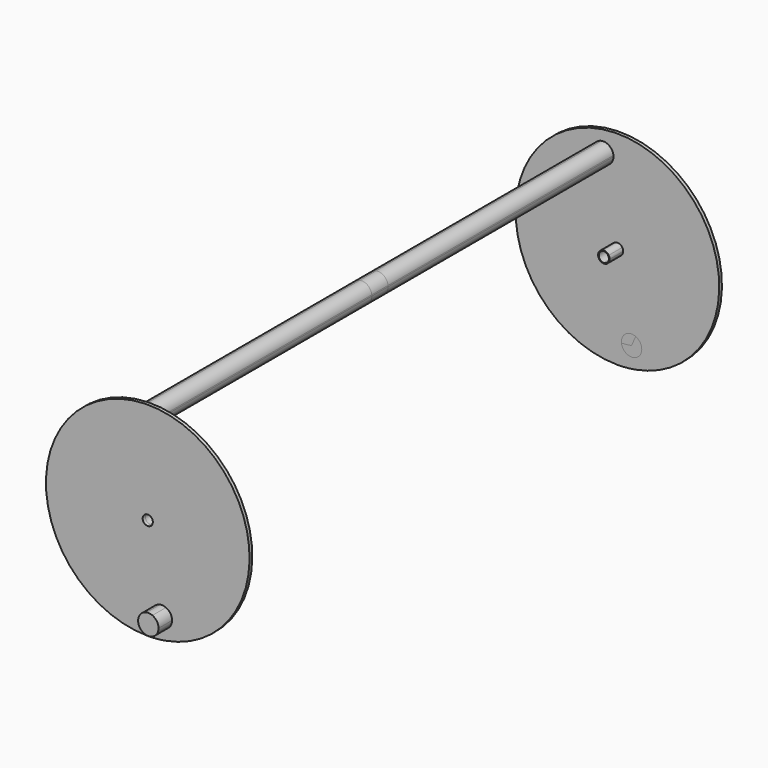
from build123d import *
from build123d import SkipClean  # not in build123d's __all__

# Parameters (mm, degrees)
F1_DEPTH = 25
F2_DEPTH = 445
F3_DEPTH = 30
F4_DEPTH = 5


# Not quite as in the source:
# - after a boolean that leaves OpenCascade's solid faulty, fix() repairs it


with BuildPart() as f1:
    # F0 (on Front) → F1 (new body)
    with BuildSketch(Plane.XZ):
        with BuildLine():
            ThreePointArc((1.4760095102, -8.3708659006), (6.5113777665, -5.4636946823), (8.5, 0))
            Line((8.5, 0), (7.5, 0))
            ThreePointArc((7.5, 0), (5.7453333234, -4.8209070726), (1.3023613325, -7.3860581476))
            Line((1.3023613325, -7.3860581476), (1.4760095102, -8.3708659006))
        make_face()
        with BuildLine():
            Line((7.5, 0), (8.5, 0))
            ThreePointArc((8.5, 0), (8.1523783886, 2.405977267), (7.1379466801, 4.6151616647))
            Line((7.1379466801, 4.6151616647), (6.2981882472, 4.0722014689))
            ThreePointArc((6.2981882472, 4.0722014689), (7.1932750487, 2.122921118), (7.5, 0))
        make_face()
        with BuildLine():
            ThreePointArc((-1.4760095102, 8.3708659006), (-8.4676549338, -0.7408238134), (0, -8.5))
            Line((0, -8.5), (0, -7.5))
            ThreePointArc((0, -7.5), (-7.4714602357, -0.6536680706), (-1.3023613325, 7.3860581476))
            Line((-1.3023613325, 7.3860581476), (-1.4760095102, 8.3708659006))
        make_face()
        with BuildLine():
            Line((0, -7.5), (0, -8.5))
            ThreePointArc((0, -8.5), (0.7408238134, -8.4676549338), (1.4760095102, -8.3708659006))
            Line((1.4760095102, -8.3708659006), (1.3023613325, -7.3860581476))
            ThreePointArc((1.3023613325, -7.3860581476), (0.6536680706, -7.4714602357), (0, -7.5))
        make_face()
        with BuildLine():
            Line((6.2981882472, 4.0722014689), (7.1379466801, 4.6151616647))
            ThreePointArc((7.1379466801, 4.6151616647), (3.397162302, 7.7916165392), (-1.4760095102, 8.3708659006))
            Line((-1.4760095102, 8.3708659006), (-1.3023613325, 7.3860581476))
            ThreePointArc((-1.3023613325, 7.3860581476), (2.9974961488, 6.8749557699), (6.2981882472, 4.0722014689))
        make_face()
    extrude(amount=-F1_DEPTH)



with BuildPart() as f2:
    # F0 (on Front) → F2 (new body)
    with BuildSketch(Plane.XZ):
        with BuildLine():
            ThreePointArc((-5.9317498787, 119.8533034312), (-11.8541755818, 130.1892085775), (-23.442503985, 132.9490466566))
            Line((-23.442503985, 132.9490466566), (-20.83778132, 118.1769303615))
            ThreePointArc((-20.83778132, 118.1769303615), (-13.4109845581, 119.2482515309), (-5.9317498787, 119.8533034312))
        make_face()
        with BuildLine():
            Line((-20.83778132, 118.1769303615), (-23.442503985, 132.9490466566))
            ThreePointArc((-23.442503985, 132.9490466566), (-33.3880504574, 126.3922054378), (-35.4182224283, 114.6540427548))
            ThreePointArc((-35.4182224283, 114.6540427548), (-28.1831008533, 116.6435288659), (-20.83778132, 118.1769303615))
        make_face()
        with BuildLine():
            ThreePointArc((-5.9317498787, 119.8533034312), (-13.4109845581, 119.2482515309), (-20.83778132, 118.1769303615))
            Line((-20.83778132, 118.1769303615), (-18.233058655, 103.4048140663))
            ThreePointArc((-18.233058655, 103.4048140663), (-9.3471146732, 108.5351162162), (-5.83778132, 118.1769303615))
            ThreePointArc((-5.83778132, 118.1769303615), (-5.8612918846, 119.016432708), (-5.9317498787, 119.8533034312))
        make_face()
        with BuildLine():
            Line((-18.233058655, 103.4048140663), (-20.83778132, 118.1769303615))
            ThreePointArc((-20.83778132, 118.1769303615), (-28.1831008533, 116.6435288659), (-35.4182224283, 114.6540427548))
            ThreePointArc((-35.4182224283, 114.6540427548), (-29.0530563964, 105.6266612241), (-18.233058655, 103.4048140663))
        make_face()
    extrude(amount=-F2_DEPTH)


with BuildPart() as f3:
    # F0 (on Front) → F3 (new body)
    with BuildSketch(Plane.XZ):
        with BuildLine():
            ThreePointArc((5.9317498787, -119.8533034312), (11.8541755818, -130.1892085775), (23.442503985, -132.9490466566))
            Line((23.442503985, -132.9490466566), (20.83778132, -118.1769303615))
            ThreePointArc((20.83778132, -118.1769303615), (13.4109845581, -119.2482515309), (5.9317498787, -119.8533034312))
        make_face()
        with BuildLine():
            Line((20.83778132, -118.1769303615), (23.442503985, -132.9490466566))
            ThreePointArc((23.442503985, -132.9490466566), (32.3284479668, -127.8187445068), (35.83778132, -118.1769303615))
            ThreePointArc((35.83778132, -118.1769303615), (35.7325222816, -116.4030386826), (35.4182224283, -114.6540427548))
            ThreePointArc((35.4182224283, -114.6540427548), (28.1831008533, -116.6435288659), (20.83778132, -118.1769303615))
        make_face()
        with BuildLine():
            ThreePointArc((20.83778132, -118.1769303615), (28.1831008533, -116.6435288659), (35.4182224283, -114.6540427548))
            ThreePointArc((35.4182224283, -114.6540427548), (32.3262590082, -108.5325081181), (26.8327736176, -104.4270188217))
            Line((26.8327736176, -104.4270188217), (20.83778132, -118.1769303615))
        make_face()
        with BuildLine():
            Line((18.233058655, -103.4048140663), (20.83778132, -118.1769303615))
            Line((20.83778132, -118.1769303615), (26.8327736176, -104.4270188217))
            ThreePointArc((26.8327736176, -104.4270188217), (22.6082918921, -103.2817871156), (18.233058655, -103.4048140663))
        make_face()
        with BuildLine():
            ThreePointArc((5.9317498787, -119.8533034312), (13.4109845581, -119.2482515309), (20.83778132, -118.1769303615))
            Line((20.83778132, -118.1769303615), (18.233058655, -103.4048140663))
            ThreePointArc((18.233058655, -103.4048140663), (8.8255031039, -109.1933246233), (5.9317498787, -119.8533034312))
        make_face()
    extrude(amount=F3_DEPTH)


with BuildPart() as f1_1:
    add(f1.part, clean=False)

    with SkipClean():  # cleaning this boolean's faces spoils the solid; the shape is the same uncleaned
        add(f2.part)  # F4 merges F2

    with SkipClean():  # cleaning this boolean's faces spoils the solid; the shape is the same uncleaned
        add(f3.part)  # F4 merges F3
    # F0 (on Front) → F4 (join)
    with BuildSketch(Plane.XZ):
        with BuildLine():
            Line((120, 0), (150, 0))
            ThreePointArc((150, 0), (143.8655009749, 42.4584223594), (125.9637649434, 81.4440293778))
            Line((125.9637649434, 81.4440293778), (113.367388449, 73.29962644))
            ThreePointArc((113.367388449, 73.29962644), (115.1575620522, 69.4010657382), (115.7710119547, 65.1552235022))
            ThreePointArc((115.7710119547, 65.1552235022), (113.7154721999, 57.5762427686), (108.11221876, 52.0744481949))
            ThreePointArc((108.11221876, 52.0744481949), (116.9903121015, 26.7070566406), (120, 0))
        make_face()
        with BuildLine():
            ThreePointArc((26.04722665, -147.7211629518), (114.9066664678, -96.418141453), (150, 0))
            Line((150, 0), (120, 0))
            ThreePointArc((120, 0), (96.5665229036, -71.2383790825), (35.4182224283, -114.6540427548))
            ThreePointArc((35.4182224283, -114.6540427548), (35.7325222816, -116.4030386826), (35.83778132, -118.1769303615))
            ThreePointArc((35.83778132, -118.1769303615), (32.3284479668, -127.8187445068), (23.442503985, -132.9490466566))
            Line((23.442503985, -132.9490466566), (26.04722665, -147.7211629518))
        make_face()
        with BuildLine():
            Line((113.367388449, 73.29962644), (125.9637649434, 81.4440293778))
            ThreePointArc((125.9637649434, 81.4440293778), (59.949922976, 137.4991153978), (-26.04722665, 147.7211629518))
            Line((-26.04722665, 147.7211629518), (-23.442503985, 132.9490466566))
            ThreePointArc((-23.442503985, 132.9490466566), (-11.8541755818, 130.1892085775), (-5.9317498787, 119.8533034312))
            ThreePointArc((-5.9317498787, 119.8533034312), (47.9599383808, 109.9992923182), (91.8552580876, 77.2179484424))
            ThreePointArc((91.8552580876, 77.2179484424), (103.4589586729, 79.9124231838), (113.367388449, 73.29962644))
        make_face()
        with BuildLine():
            ThreePointArc((0, -150), (13.0733614121, -149.4292047138), (26.04722665, -147.7211629518))
            Line((26.04722665, -147.7211629518), (23.442503985, -132.9490466566))
            ThreePointArc((23.442503985, -132.9490466566), (11.8541755818, -130.1892085775), (5.9317498787, -119.8533034312))
            ThreePointArc((5.9317498787, -119.8533034312), (2.9667817794, -119.963320252), (0, -120))
            Line((0, -120), (0, -150))
        make_face()
        with BuildLine():
            ThreePointArc((35.4182224283, -114.6540427548), (96.5665229036, -71.2383790825), (120, 0))
            Line((120, 0), (72.3631882451, 0))
            Line((72.3631882451, 0), (26.8327736176, -104.4270188217))
            ThreePointArc((26.8327736176, -104.4270188217), (32.3262590082, -108.5325081181), (35.4182224283, -114.6540427548))
        make_face()
        with BuildLine():
            Line((72.3631882451, 0), (120, 0))
            ThreePointArc((120, 0), (116.9903121015, 26.7070566406), (108.11221876, 52.0744481949))
            ThreePointArc((108.11221876, 52.0744481949), (101.522682893, 50.1740689806), (94.7760196571, 51.4053119625))
            Line((94.7760196571, 51.4053119625), (72.3631882451, 0))
        make_face()
        with BuildLine():
            Line((-23.442503985, 132.9490466566), (-26.04722665, 147.7211629518))
            ThreePointArc((-26.04722665, 147.7211629518), (-149.4292047138, -13.0733614122), (0, -150))
            Line((0, -150), (0, -120))
            ThreePointArc((0, -120), (-118.6559841107, -17.9097022508), (-35.4182224283, 114.6540427548))
            ThreePointArc((-35.4182224283, 114.6540427548), (-33.3880504574, 126.3922054378), (-23.442503985, 132.9490466566))
        make_face()
        with BuildLine():
            ThreePointArc((115.7710119547, 65.1552235022), (115.1575620522, 69.4010657382), (113.367388449, 73.29962644))
            Line((113.367388449, 73.29962644), (100.7710119547, 65.1552235022))
            ThreePointArc((100.7710119547, 65.1552235022), (104.6462024591, 58.7296544421), (108.11221876, 52.0744481949))
            ThreePointArc((108.11221876, 52.0744481949), (113.7154721999, 57.5762427686), (115.7710119547, 65.1552235022))
        make_face()
        with BuildLine():
            Line((100.7710119547, 65.1552235022), (113.367388449, 73.29962644))
            ThreePointArc((113.367388449, 73.29962644), (103.4589586729, 79.9124231838), (91.8552580876, 77.2179484424))
            ThreePointArc((91.8552580876, 77.2179484424), (96.5017995213, 71.3260309365), (100.7710119547, 65.1552235022))
        make_face()
        with BuildLine():
            Line((26.8327736176, -104.4270188217), (72.3631882451, 0))
            Line((72.3631882451, 0), (8.5, 0))
            ThreePointArc((8.5, 0), (6.5113777665, -5.4636946823), (1.4760095102, -8.3708659006))
            Line((1.4760095102, -8.3708659006), (18.233058655, -103.4048140663))
            ThreePointArc((18.233058655, -103.4048140663), (22.6082918921, -103.2817871156), (26.8327736176, -104.4270188217))
        make_face()
        with BuildLine():
            Line((8.5, 0), (72.3631882451, 0))
            Line((72.3631882451, 0), (94.7760196571, 51.4053119625))
            ThreePointArc((94.7760196571, 51.4053119625), (91.0619862538, 53.7212906732), (88.1746354604, 57.0108205645))
            Line((88.1746354604, 57.0108205645), (7.1379466801, 4.6151616647))
            ThreePointArc((7.1379466801, 4.6151616647), (8.1523783886, 2.405977267), (8.5, 0))
        make_face()
        with BuildLine():
            ThreePointArc((94.7760196571, 51.4053119625), (101.522682893, 50.1740689806), (108.11221876, 52.0744481949))
            ThreePointArc((108.11221876, 52.0744481949), (104.6462024591, 58.7296544421), (100.7710119547, 65.1552235022))
            Line((100.7710119547, 65.1552235022), (94.7760196571, 51.4053119625))
        make_face()
        with BuildLine():
            ThreePointArc((-5.9317498787, 119.8533034312), (-11.8541755818, 130.1892085775), (-23.442503985, 132.9490466566))
            Line((-23.442503985, 132.9490466566), (-20.83778132, 118.1769303615))
            ThreePointArc((-20.83778132, 118.1769303615), (-13.4109845581, 119.2482515309), (-5.9317498787, 119.8533034312))
        make_face()
        with BuildLine():
            Line((-20.83778132, 118.1769303615), (-23.442503985, 132.9490466566))
            ThreePointArc((-23.442503985, 132.9490466566), (-33.3880504574, 126.3922054378), (-35.4182224283, 114.6540427548))
            ThreePointArc((-35.4182224283, 114.6540427548), (-28.1831008533, 116.6435288659), (-20.83778132, 118.1769303615))
        make_face()
        with BuildLine():
            Line((94.7760196571, 51.4053119625), (100.7710119547, 65.1552235022))
            Line((100.7710119547, 65.1552235022), (88.1746354604, 57.0108205645))
            ThreePointArc((88.1746354604, 57.0108205645), (91.0619862538, 53.7212906732), (94.7760196571, 51.4053119625))
        make_face()
        with BuildLine():
            Line((88.1746354604, 57.0108205645), (100.7710119547, 65.1552235022))
            ThreePointArc((100.7710119547, 65.1552235022), (96.5017995213, 71.3260309365), (91.8552580876, 77.2179484424))
            ThreePointArc((91.8552580876, 77.2179484424), (86.0138122732, 67.8431702204), (88.1746354604, 57.0108205645))
        make_face()
        with BuildLine():
            ThreePointArc((88.1746354604, 57.0108205645), (86.0138122732, 67.8431702204), (91.8552580876, 77.2179484424))
            ThreePointArc((91.8552580876, 77.2179484424), (47.9599383808, 109.9992923182), (-5.9317498787, 119.8533034312))
            ThreePointArc((-5.9317498787, 119.8533034312), (-5.8612918846, 119.016432708), (-5.83778132, 118.1769303615))
            ThreePointArc((-5.83778132, 118.1769303615), (-9.3471146732, 108.5351162162), (-18.233058655, 103.4048140663))
            Line((-18.233058655, 103.4048140663), (-1.4760095102, 8.3708659006))
            ThreePointArc((-1.4760095102, 8.3708659006), (3.397162302, 7.7916165392), (7.1379466801, 4.6151616647))
            Line((7.1379466801, 4.6151616647), (88.1746354604, 57.0108205645))
        make_face()
        with BuildLine():
            ThreePointArc((-35.4182224283, 114.6540427548), (-118.6559841107, -17.9097022508), (0, -120))
            Line((0, -120), (0, -8.5))
            ThreePointArc((0, -8.5), (-8.4676549338, -0.7408238134), (-1.4760095102, 8.3708659006))
            Line((-1.4760095102, 8.3708659006), (-18.233058655, 103.4048140663))
            ThreePointArc((-18.233058655, 103.4048140663), (-29.0530563964, 105.6266612241), (-35.4182224283, 114.6540427548))
        make_face()
        with BuildLine():
            Line((0, -8.5), (0, -120))
            ThreePointArc((0, -120), (2.9667817794, -119.963320252), (5.9317498787, -119.8533034312))
            ThreePointArc((5.9317498787, -119.8533034312), (8.8255031039, -109.1933246233), (18.233058655, -103.4048140663))
            Line((18.233058655, -103.4048140663), (1.4760095102, -8.3708659006))
            ThreePointArc((1.4760095102, -8.3708659006), (0.7408238134, -8.4676549338), (0, -8.5))
        make_face()
        with BuildLine():
            Line((18.233058655, -103.4048140663), (20.83778132, -118.1769303615))
            Line((20.83778132, -118.1769303615), (26.8327736176, -104.4270188217))
            ThreePointArc((26.8327736176, -104.4270188217), (22.6082918921, -103.2817871156), (18.233058655, -103.4048140663))
        make_face()
        with BuildLine():
            ThreePointArc((5.9317498787, -119.8533034312), (13.4109845581, -119.2482515309), (20.83778132, -118.1769303615))
            Line((20.83778132, -118.1769303615), (18.233058655, -103.4048140663))
            ThreePointArc((18.233058655, -103.4048140663), (8.8255031039, -109.1933246233), (5.9317498787, -119.8533034312))
        make_face()
        with BuildLine():
            ThreePointArc((1.4760095102, -8.3708659006), (6.5113777665, -5.4636946823), (8.5, 0))
            Line((8.5, 0), (7.5, 0))
            ThreePointArc((7.5, 0), (5.7453333234, -4.8209070726), (1.3023613325, -7.3860581476))
            Line((1.3023613325, -7.3860581476), (1.4760095102, -8.3708659006))
        make_face()
        with BuildLine():
            Line((7.5, 0), (8.5, 0))
            ThreePointArc((8.5, 0), (8.1523783886, 2.405977267), (7.1379466801, 4.6151616647))
            Line((7.1379466801, 4.6151616647), (6.2981882472, 4.0722014689))
            ThreePointArc((6.2981882472, 4.0722014689), (7.1932750487, 2.122921118), (7.5, 0))
        make_face()
        with BuildLine():
            ThreePointArc((-5.9317498787, 119.8533034312), (-13.4109845581, 119.2482515309), (-20.83778132, 118.1769303615))
            Line((-20.83778132, 118.1769303615), (-18.233058655, 103.4048140663))
            ThreePointArc((-18.233058655, 103.4048140663), (-9.3471146732, 108.5351162162), (-5.83778132, 118.1769303615))
            ThreePointArc((-5.83778132, 118.1769303615), (-5.8612918846, 119.016432708), (-5.9317498787, 119.8533034312))
        make_face()
        with BuildLine():
            Line((-18.233058655, 103.4048140663), (-20.83778132, 118.1769303615))
            ThreePointArc((-20.83778132, 118.1769303615), (-28.1831008533, 116.6435288659), (-35.4182224283, 114.6540427548))
            ThreePointArc((-35.4182224283, 114.6540427548), (-29.0530563964, 105.6266612241), (-18.233058655, 103.4048140663))
        make_face()
        with BuildLine():
            ThreePointArc((-1.4760095102, 8.3708659006), (-8.4676549338, -0.7408238134), (0, -8.5))
            Line((0, -8.5), (0, -7.5))
            ThreePointArc((0, -7.5), (-7.4714602357, -0.6536680706), (-1.3023613325, 7.3860581476))
            Line((-1.3023613325, 7.3860581476), (-1.4760095102, 8.3708659006))
        make_face()
        with BuildLine():
            Line((0, -7.5), (0, -8.5))
            ThreePointArc((0, -8.5), (0.7408238134, -8.4676549338), (1.4760095102, -8.3708659006))
            Line((1.4760095102, -8.3708659006), (1.3023613325, -7.3860581476))
            ThreePointArc((1.3023613325, -7.3860581476), (0.6536680706, -7.4714602357), (0, -7.5))
        make_face()
        with BuildLine():
            Line((6.2981882472, 4.0722014689), (7.1379466801, 4.6151616647))
            ThreePointArc((7.1379466801, 4.6151616647), (3.397162302, 7.7916165392), (-1.4760095102, 8.3708659006))
            Line((-1.4760095102, 8.3708659006), (-1.3023613325, 7.3860581476))
            ThreePointArc((-1.3023613325, 7.3860581476), (2.9974961488, 6.8749557699), (6.2981882472, 4.0722014689))
        make_face()
    with SkipClean():  # cleaning this boolean's faces spoils the solid; the shape is the same uncleaned
        extrude(amount=F4_DEPTH)

    # F6: F1 across plane


with BuildPart() as f1_2:
    add(f1_1.part, clean=False)
    add(f1_1.part.mirror(Plane.XZ.offset(-430)), clean=False)

    add(f1_2.part.fix(), mode=Mode.REPLACE)


solid = f1_2.part
